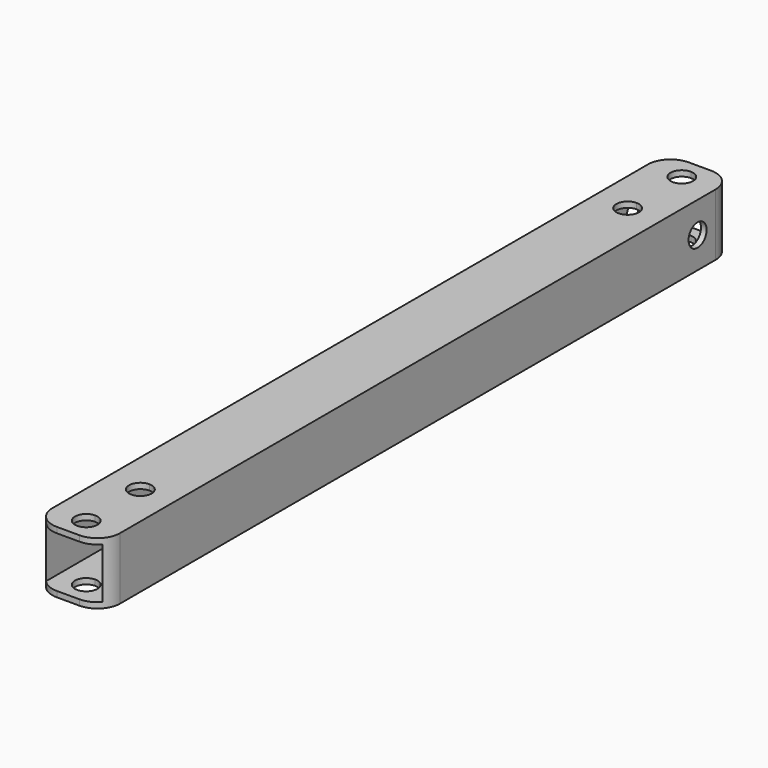
from build123d import *

# Parameters (mm, degrees)
F0_W        = 30
F0_H        = 27.5
F0_W_2      = 25
F0_H_2      = 22.5
F1_DEPTH    = 350
F3_DEPTH    = 53
F4_T1_DEPTH = 77.5
F5_R        = 5
F6_DEPTH    = 37.8


# Not quite as in the source:
# - a fillet or chamfer that OpenCascade refuses, or shapes differently, is made with other operations: its cross-section is extruded or revolved along the edge and cut away or added
# - a feature names something its author has since deleted; it is built from what else it names


with BuildPart() as f1:
    # F0 (on Front) → F1 (new body)
    with BuildSketch(Plane.XZ):
        with Locations((-59.9858543277, 13.75)):
            Rectangle(F0_W, F0_H)
        with Locations((-59.9858543277, 13.75)):
            Rectangle(F0_W_2, F0_H_2, mode=Mode.SUBTRACT)
    extrude(amount=F1_DEPTH)

    # F2 (on Top) → F3 (cut)
    with BuildSketch(Plane.XY):
        with BuildLine():
            Line((-59.9858543277, -340), (-59.9858543277, -335))
            ThreePointArc((-59.9858543277, -335), (-64.9858543277, -340), (-59.9858543277, -345))
            Line((-59.9858543277, -345), (-59.9858543277, -340))
        make_face()
        with BuildLine():
            ThreePointArc((-54.9858543277, -340), (-56.4503204217, -336.4644660941), (-59.9858543277, -335))
            Line((-59.9858543277, -335), (-59.9858543277, -340))
            Line((-59.9858543277, -340), (-59.9858543277, -345))
            ThreePointArc((-59.9858543277, -345), (-56.4503204217, -343.5355339059), (-54.9858543277, -340))
        make_face()
        with BuildLine():
            Line((-59.9858543277, -45), (-59.9858543277, -35))
            ThreePointArc((-59.9858543277, -35), (-64.9858543277, -40), (-59.9858543277, -45))
        make_face()
        with BuildLine():
            ThreePointArc((-54.9858543277, -40), (-56.4503204217, -36.4644660941), (-59.9858543277, -35))
            Line((-59.9858543277, -35), (-59.9858543277, -45))
            ThreePointArc((-59.9858543277, -45), (-56.4503204217, -43.5355339059), (-54.9858543277, -40))
        make_face()
        with BuildLine():
            Line((-59.9858543277, -15), (-59.9858543277, -5))
            ThreePointArc((-59.9858543277, -5), (-64.9858543277, -10), (-59.9858543277, -15))
        make_face()
        with BuildLine():
            ThreePointArc((-59.9858543277, -15), (-56.4503204217, -13.5355339059), (-54.9858543277, -10))
            ThreePointArc((-54.9858543277, -10), (-56.4503204217, -6.4644660941), (-59.9858543277, -5))
            Line((-59.9858543277, -5), (-59.9858543277, -15))
        make_face()
        with BuildLine():
            Line((-59.9858543277, -315), (-59.9858543277, -305))
            ThreePointArc((-59.9858543277, -305), (-64.9858543277, -310), (-59.9858543277, -315))
        make_face()
        with BuildLine():
            ThreePointArc((-54.9858543277, -310), (-56.4503204217, -306.4644660941), (-59.9858543277, -305))
            Line((-59.9858543277, -305), (-59.9858543277, -315))
            ThreePointArc((-59.9858543277, -315), (-56.4503204217, -313.5355339059), (-54.9858543277, -310))
        make_face()
    extrude(amount=F3_DEPTH, mode=Mode.SUBTRACT)

    # F4: fillet of radius 10 on 4 edges, made by hand

    # F4_s2 → F4_t1 (cut)
    with BuildSketch(Plane.XY.offset(-25)):
        with BuildLine():
            ThreePointArc((-74.9858543277, -10), (-72.0569221395, -2.9289321881), (-64.9858543277, 0))
            Line((-64.9858543277, 0), (-74.9858543277, 0))
            Line((-74.9858543277, 0), (-74.9858543277, -10))
        make_face()
        with BuildLine():
            ThreePointArc((-74.9858543277, -340), (-72.0569221395, -347.0710678119), (-64.9858543277, -350))
            Line((-64.9858543277, -350), (-74.9858543277, -350))
            Line((-74.9858543277, -350), (-74.9858543277, -340))
        make_face()
        with BuildLine():
            ThreePointArc((-54.9858543277, 0), (-47.9147865158, -2.9289321881), (-44.9858543277, -10))
            Line((-44.9858543277, -10), (-44.9858543277, 0))
            Line((-44.9858543277, 0), (-54.9858543277, 0))
        make_face()
        with BuildLine():
            ThreePointArc((-54.9858543277, -350), (-47.9147865158, -347.0710678119), (-44.9858543277, -340))
            Line((-44.9858543277, -340), (-44.9858543277, -350))
            Line((-44.9858543277, -350), (-54.9858543277, -350))
        make_face()
    extrude(amount=F4_T1_DEPTH, mode=Mode.SUBTRACT)

    # F5 (on face) → F6 (cut)
    with BuildSketch(Plane.YZ.offset(-44.9858543277)):
        with Locations((-20, 13.75)):
            Circle(F5_R)
    extrude(amount=-F6_DEPTH, mode=Mode.SUBTRACT)


solid = f1.part
